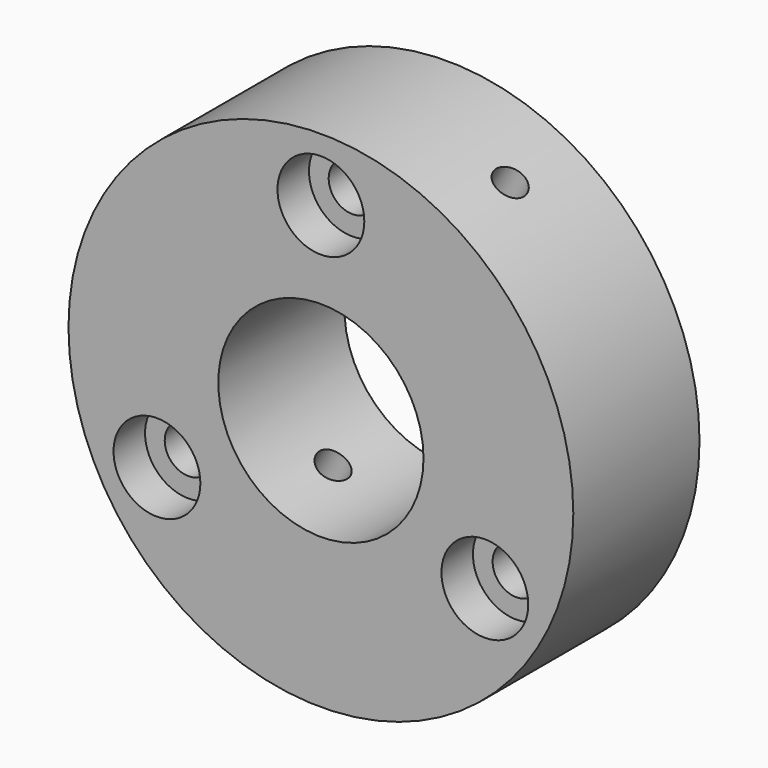
from build123d import *

# Parameters (mm, degrees)
F0_R           = 25.4
F0_R_2         = 10.3251
F1_DEPTH       = 15.875
F3_D           = 4.7752
F3_CBORE_D     = 8.7376
F3_CBORE_DEPTH = 3.9624
F6_R           = 1.5875
F7_DEPTH       = 9.2980452561
F8_R           = 1.5875
F9_DEPTH       = 60.0980452561


with BuildPart() as f1:
    # F0 (on Front) → F1 (new body)
    with BuildSketch(Plane.XZ):
        Circle(F0_R)
        Circle(F0_R_2, mode=Mode.SUBTRACT)
    extrude(amount=F1_DEPTH)

    # F3 (through all)
    with Locations(Plane.XZ.offset(15.875)):
        with Locations((0, 19.05), (-16.4977839421, -9.525), (16.4977839421, -9.525)):
            CounterBoreHole(F3_D / 2, F3_CBORE_D / 2, F3_CBORE_DEPTH)

    # F6 (on face) → F7 (cut, through all)
    with BuildSketch(Plane(origin=(12.7, 0, 21.9970452561), x_dir=(0.8660254038, 0, -0.5), z_dir=(-0.5, 0, -0.8660254038))):
        with Locations((0.8242388722, 7.9502)):
            Circle(F6_R)
    extrude(amount=-F7_DEPTH, mode=Mode.SUBTRACT)

    # F8 (on face) → F9 (cut, through all)
    with BuildSketch(Plane(origin=(12.7, 0, 21.9970452561), x_dir=(0.8660254038, 0, -0.5), z_dir=(-0.5, 0, -0.8660254038))):
        with Locations((0, 7.9248)):
            Circle(F8_R)
    extrude(amount=F9_DEPTH, mode=Mode.SUBTRACT)


solid = f1.part
